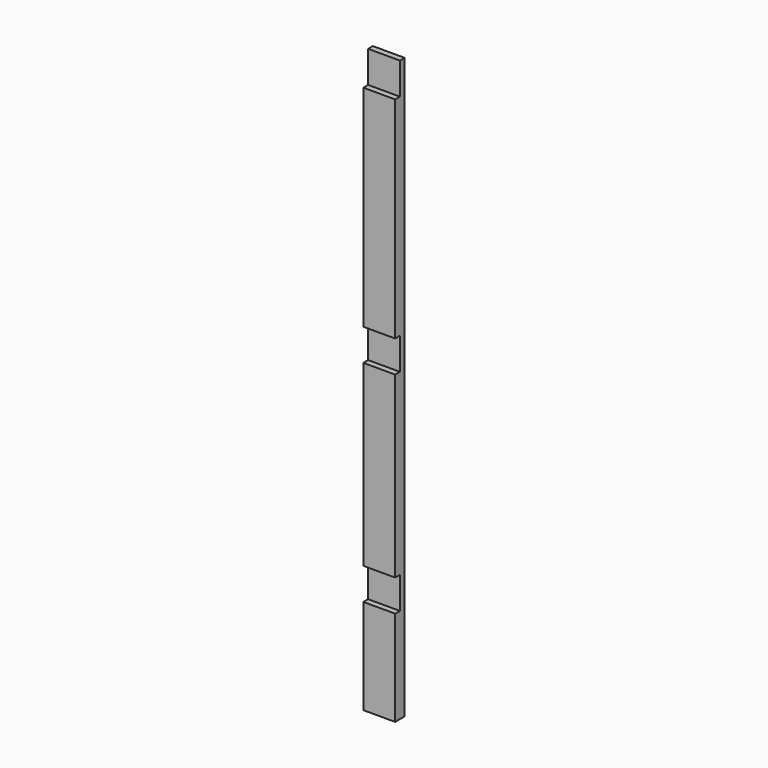
from build123d import *

# Parameters (mm, degrees)
F0_W     = 50.8
F0_H     = 19.05
F1_DEPTH = 927.1
F2_W     = 122.43557321
F2_H     = 50.8
F2_W_2   = 343.1604206562
F2_W_3   = 264.5317912102
F3_DEPTH = 25.4


# Not quite as in the source:
# - a feature names something its author has since deleted; it is built from what else it names


with BuildPart() as f1:
    # F0 (on Top) → F1 (new body)
    with BuildSketch(Plane.XY):
        Rectangle(F0_W, F0_H)
    extrude(amount=F1_DEPTH)

    # F2 (on Front) → F3 (cut)
    with BuildSketch(Plane.XZ):
        with Locations((22.4465244144, 177.8)):
            Rectangle(F2_W, F2_H)
        with Locations((-38.7818217278, 901.7)):
            Rectangle(F2_W_2, F2_H)
        with Locations((-47.6498156786, 514.35)):
            Rectangle(F2_W_3, F2_H)
    extrude(amount=F3_DEPTH, mode=Mode.SUBTRACT)


solid = f1.part
